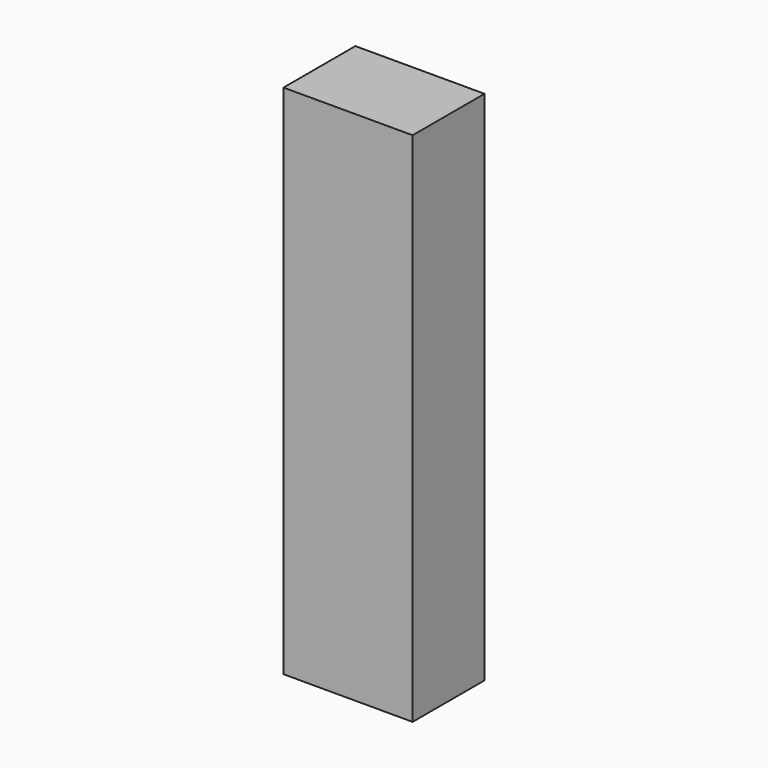
from build123d import *

# Parameters (mm, degrees)
F0_W     = 146.05
F0_H     = 101.6
F1_DEPTH = 584.2


# Not quite as in the source:
# - the program builds the solid bodies; features that only make, move or delete a surface that nothing else refers to are left out


with BuildPart() as f1:
    # F0 (on Top) → F1 (new body)
    with BuildSketch(Plane.XY):
        Rectangle(F0_W, F0_H)
    extrude(amount=F1_DEPTH)


solid = f1.part
